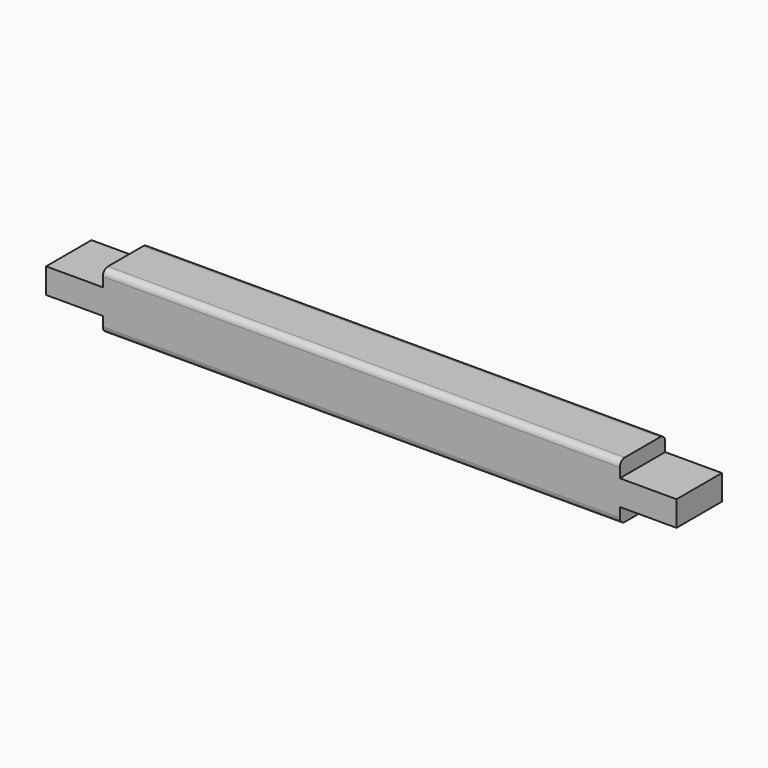
from build123d import *

# Parameters (mm, degrees)
F0_W     = 45
F0_H     = 45
F1_DEPTH = 250
F2_R     = 5
F3_W     = 45
F3_H     = 12.5
F4_DEPTH = 45.001
F5_W     = 40
F5_H     = 20
F6_DEPTH = 25
F7_W     = 40
F7_H     = 20
F8_DEPTH = 25


# Not quite as in the source:
# - a pattern or mirror of a feature is missing from the dataset's text; its kind, count and spacing are read off the source's solid


with BuildPart() as f1:
    # F0 (on Right) → F1 (new body, symmetric)
    with BuildSketch(Plane.YZ):
        with Locations((22.5, 22.5)):
            Rectangle(F0_W, F0_H)
    extrude(amount=F1_DEPTH, both=True)

    # F2
    f2_edges = [f1.edges().sort_by_distance(p)[0] for p in [
        (0, 0, 45),
        (0, 45, 45),
        (0, 0, 0),
        (0, 45, 0),
    ]]
    fillet(f2_edges, radius=F2_R)

    # F3 (on face) → F4 (cut, through all)
    with BuildSketch(Plane.XZ):
        with Locations((-227.5, 6.25)):
            Rectangle(F3_W, F3_H)
        with Locations((-227.5, 38.75)):
            Rectangle(F3_W, F3_H)
    f4 = extrude(amount=-F4_DEPTH, mode=Mode.SUBTRACT)

    # F4_copies: F4 across plane
    add(f4.mirror(Plane(origin=(0, 0, 0), x_dir=(0, 0, 1), z_dir=(1, 0, 0))), mode=Mode.SUBTRACT)

    # F5 (on face) → F6 (cut)
    with BuildSketch(Plane(origin=(-250, 0, 0), x_dir=(0, -1, 0), z_dir=(-1, 0, 0))):
        with Locations((150, 22.5)):
            Rectangle(F5_W, F5_H)
    extrude(amount=-F6_DEPTH, mode=Mode.SUBTRACT)

    # F7 (on face) → F8 (cut)
    with BuildSketch(Plane(origin=(0, 0, 0), x_dir=(1, 0, 0), z_dir=(0, 0, -1))):
        with Locations((-80, -22.5)):
            Rectangle(F7_W, F7_H)
    f8 = extrude(amount=-F8_DEPTH, mode=Mode.SUBTRACT)

    # F8_copies: F8 across plane
    add(f8.mirror(Plane(origin=(0, 0, 0), x_dir=(0, 0, 1), z_dir=(1, 0, 0))), mode=Mode.SUBTRACT)


solid = f1.part
